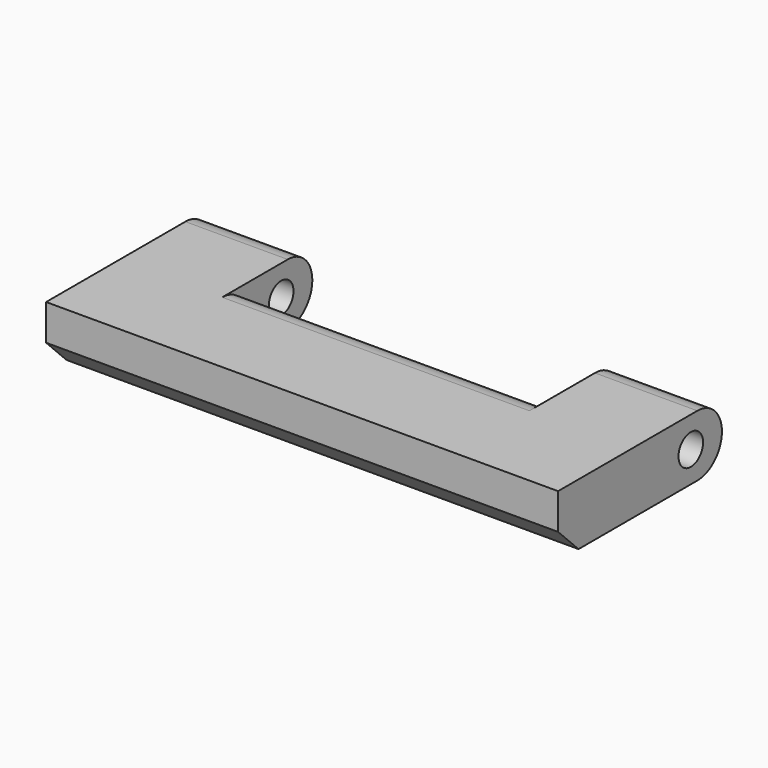
from build123d import *

# Parameters (mm, degrees)
F1_DEPTH = 6
F2_R     = 1.5
F3_DEPTH = 50.001
F4_R     = 2.99999
F5_SIZE  = 2.5


# Not quite as in the source:
# - a fillet or chamfer is up to 0.001 mm smaller than in the source, because OpenCascade refuses the exact size


with BuildPart() as f1:
    # F0 (on Top) → F1 (new body)
    with BuildSketch(Plane.XY):
        Polygon((0, 0), (0, -20), (50, -20), (50, 0), (40, 0), (40, -8), (10, -8), (10, 0), align=None)
    extrude(amount=F1_DEPTH)

    # F2 (on face) → F3 (cut, through all)
    with BuildSketch(Plane(origin=(0, 0, 0), x_dir=(0, -1, 0), z_dir=(-1, 0, 0))):
        with Locations((3.8, 3)):
            Circle(F2_R)
    extrude(amount=-F3_DEPTH, mode=Mode.SUBTRACT)

    # F4 (radius 3 in the source; OpenCascade refuses exactly that, so slightly less here)
    f4_edges = [f1.edges().sort_by_distance(p)[0] for p in [
        (5, 0, 6),
        (5, 0, 0),
        (45, 0, 6),
        (45, 0, 0),
        (25, -8, 6),
        (25, -8, 0),
    ]]
    fillet(f4_edges, radius=F4_R)

    # F5
    f5_edges = [f1.edges().sort_by_distance(p)[0] for p in [
        (25, -20, 0),
    ]]
    chamfer(f5_edges, length=F5_SIZE)


solid = f1.part
